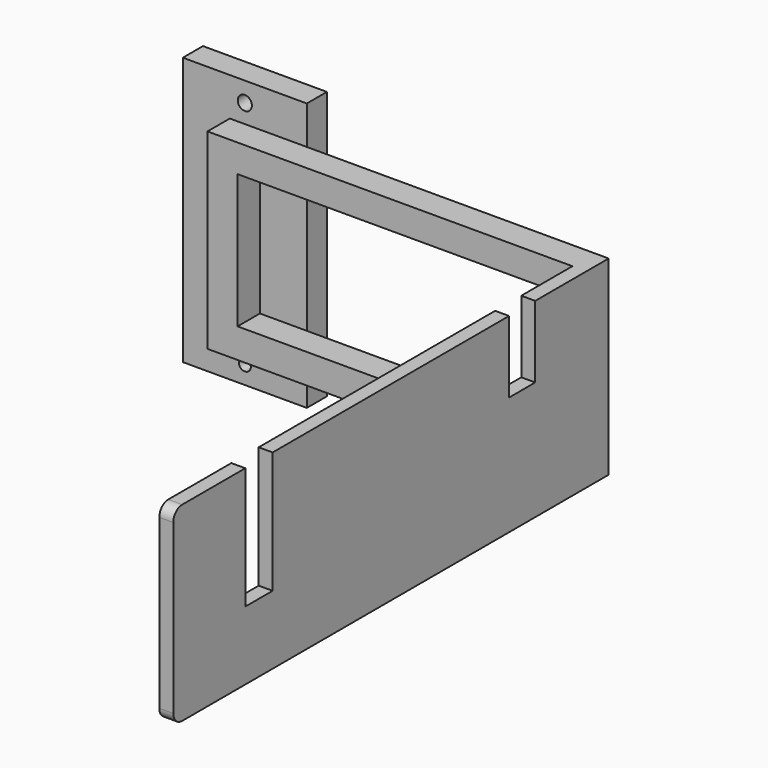
from build123d import *

# Parameters (mm, degrees)
F0_W      = 56.428283453
F0_H      = 121.9848245382
F1_DEPTH  = 6.35
F2_W      = 13.6921107769
F2_H      = 87.1320217848
F3_DEPTH  = 12.7
F4_W      = 12.7
F4_H      = 12.6656033099
F5_DEPTH  = 152.4
F6_W      = 12.7
F6_H      = 13.4637728333
F7_DEPTH  = 152.4
F8_R      = 3.224201557
F8_R_2    = 2.7149600872
F9_DEPTH  = 6.351
F10_W     = 247.7097766638
F10_H     = 86.6629034281
F11_DEPTH = 6.35
F12_W     = 14.8840993643
F12_H     = 44.3546175957
F12_W_2   = 15.5743807554
F12_H_2   = 78.4596502781
F13_DEPTH = 25.4
F14_R     = 5.08
F15_DEPTH = 5.08


# Not quite as in the source:
# - the program builds the solid bodies; features that only make, move or delete a surface that nothing else refers to are left out


with BuildPart() as f1:
    # F0 (on Front) → F1 (new body)
    with BuildSketch(Plane.XZ):
        Rectangle(F0_W, F0_H)
    extrude(amount=F1_DEPTH)

    # F2 (on face) → F3 (join)
    with BuildSketch(Plane.XZ.offset(6.35)):
        Rectangle(F2_W, F2_H)
    extrude(amount=F3_DEPTH)

    # F4 (on face) → F5 (join)
    with BuildSketch(Plane.YZ.offset(6.8460553885)):
        with Locations((-12.7, 37.2332092375)):
            Rectangle(F4_W, F4_H)
    extrude(amount=F5_DEPTH)

    # F6 (on face) → F7 (join)
    with BuildSketch(Plane.YZ.offset(6.8460553885)):
        with Locations((-12.7, -36.8341244757)):
            Rectangle(F6_W, F6_H)
    extrude(amount=F7_DEPTH)

    # F8 (on face) → F9 (cut, through all)
    with BuildSketch(Plane.XZ.offset(6.35)):
        with Locations((0, 52.0230680704)):
            Circle(F8_R)
        with Locations((0, -52.8460629284)):
            Circle(F8_R_2)
    extrude(amount=-F9_DEPTH, mode=Mode.SUBTRACT)

    # F10 (on face) → F11 (join)
    with BuildSketch(Plane.YZ.offset(159.2460553885)):
        with Locations((-130.2048883319, 0.2345591784)):
            Rectangle(F10_W, F10_H)
    extrude(amount=F11_DEPTH)

    # F12 (on face) → F13 (cut)
    with BuildSketch(Plane.YZ.offset(165.5960553885)):
        with Locations((-55.5786713958, 33.0530032516)):
            Rectangle(F12_W, F12_H)
        with Locations((-205.3182795644, 27.350962162)):
            Rectangle(F12_W_2, F12_H_2)
    extrude(amount=-F13_DEPTH, mode=Mode.SUBTRACT)

    # F14
    f14_edges = [f1.edges().sort_by_distance(p)[0] for p in [
        (162.421055, -254.059777, 43.566011),
        (162.421055, -254.059777, -43.096893),
    ]]
    fillet(f14_edges, radius=F14_R)

    # F15 (add): a face of the model
    f15_faces = [f1.faces().sort_by_distance(p)[0] for p in [
        (0, 0, -0.0696069338),
    ]]
    extrude(f15_faces, amount=F15_DEPTH)


solid = f1.part
